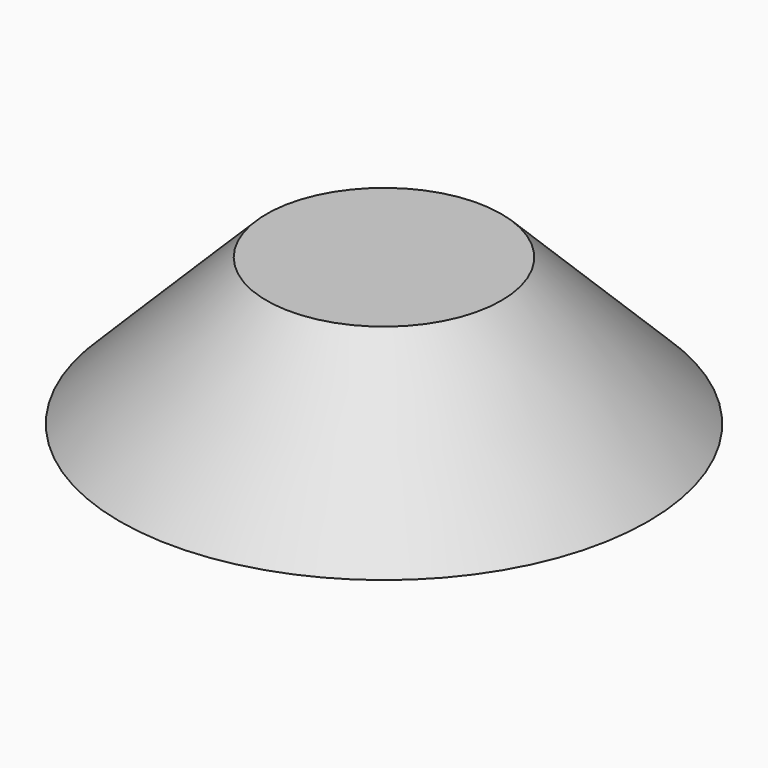
from build123d import *

# Parameters (mm, degrees)
F2_R     = 9
F3_DEPTH = 5
F4_SIZE  = 4.99999


# Not quite as in the source:
# - a fillet or chamfer is up to 0.001 mm smaller than in the source, because OpenCascade refuses the exact size
# - a feature of the source that left no trace in its solid (it failed there, or was rolled back) is left out
# - the program builds the solid bodies; features that only make, move or delete a surface that nothing else refers to are left out


with BuildPart() as f3:
    # F2 (on Top) → F3 (new body)
    with BuildSketch(Plane.XY):
        Circle(F2_R)
    extrude(amount=F3_DEPTH)

    # F4 (size 5 in the source; OpenCascade refuses exactly that, so slightly less here)
    f4_edges = [f3.edges().sort_by_distance(p)[0] for p in [
        (-9, 0, 5),
    ]]
    chamfer(f4_edges, length=F4_SIZE)


solid = f3.part
